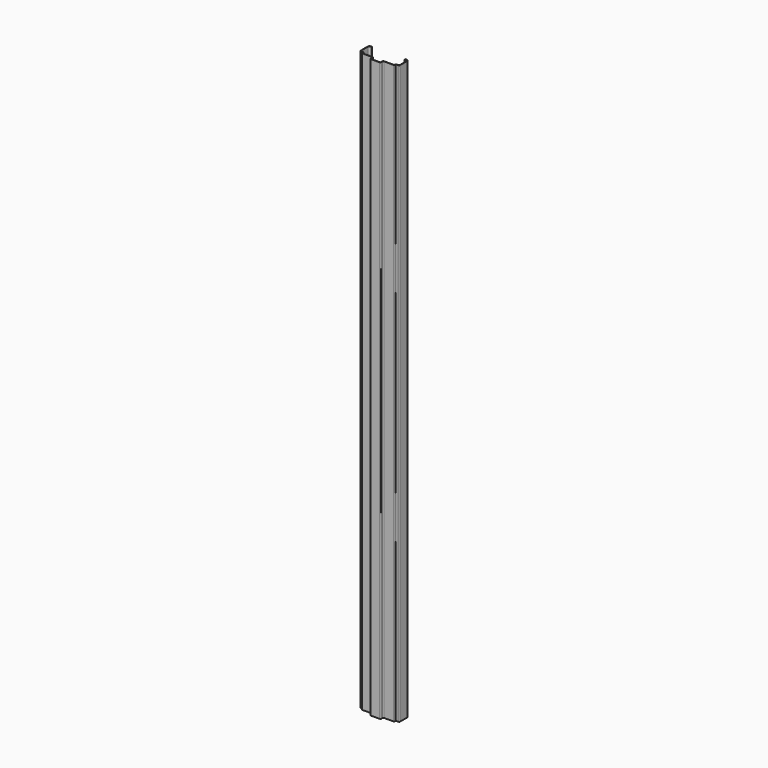
from build123d import *

# Parameters (mm, degrees)
F1_DEPTH     = 2070
F2_T1_DEPTH  = 2070
F2_T3_DEPTH  = 2070
F2_T5_DEPTH  = 2070
F2_T7_DEPTH  = 2070
F2_T9_DEPTH  = 2070
F2_T11_DEPTH = 2070
F2_T13_DEPTH = 2070
F2_T15_DEPTH = 2070
F2_T17_DEPTH = 2070
F2_T19_DEPTH = 2070
F2_T21_DEPTH = 2070
F2_T23_DEPTH = 2070
F2_T25_DEPTH = 2085
F2_T27_DEPTH = 2085
F2_T29_DEPTH = 2085
F2_T31_DEPTH = 2085
F2_T33_DEPTH = 2085
F2_T35_DEPTH = 2085
F2_T37_DEPTH = 2085
F2_T39_DEPTH = 2085
F2_T41_DEPTH = 2085
F2_T43_DEPTH = 2085
F2_T45_DEPTH = 2085
F2_T47_DEPTH = 2085
F3_R         = 5


# Not quite as in the source:
# - a fillet or chamfer that OpenCascade refuses, or shapes differently, is made with other operations: its cross-section is extruded or revolved along the edge and cut away or added


with BuildPart() as f1:
    # F0 (on Top) → F1 (new body)
    with BuildSketch(Plane.XY):
        Polygon((-18.5, 0), (0, 0), (18.5, 0), (18.5, 12), (58.5, 12), (58.5, 19), (70.5, 19), (70.5, 60), (58.5, 60), (58.5, 57), (59.5, 57), (59.5, 59), (69.5, 59), (69.5, 20), (57.5, 20), (57.5, 13), (17.5, 13), (17.5, 1), (0, 1), (-17.5, 1), (-17.5, 13), (-57.5, 13), (-57.5, 20), (-69.5, 20), (-69.5, 59), (-59.5, 59), (-59.5, 57), (-58.5, 57), (-58.5, 60), (-70.5, 60), (-70.5, 19), (-58.5, 19), (-58.5, 12), (-18.5, 12), align=None)
    extrude(amount=F1_DEPTH)

    # F2: fillet of radius 3 on 24 edges, made by hand

    # F2_s2 → F2_t1 (join)
    with BuildSketch(Plane.XY):
        with BuildLine():
            add(Edge.make_bspline(
                [(-21.5, 12), (-18.5, 12), (-18.5, 9)],
                knots=[0, 0, 0, 1, 1, 1], degree=2, weights=[1, 1, 1]))
            Line((-18.5, 9), (-18.5, 12))
            Line((-18.5, 12), (-21.5, 12))
        make_face()
    extrude(amount=F2_T1_DEPTH)

    # F2_s4 → F2_t3 (join)
    with BuildSketch(Plane.XY):
        with BuildLine():
            add(Edge.make_bspline(
                [(-61.5, 19), (-58.5, 19), (-58.5, 16)],
                knots=[0, 0, 0, 1, 1, 1], degree=2, weights=[1, 1, 1]))
            Line((-58.5, 16), (-58.5, 19))
            Line((-58.5, 19), (-61.5, 19))
        make_face()
    extrude(amount=F2_T3_DEPTH)

    # F2_s6 → F2_t5 (join)
    with BuildSketch(Plane.XY):
        with BuildLine():
            add(Edge.make_bspline(
                [(-62.3284271247, 59), (-60.2071067812, 59), (-59.5, 57)],
                knots=[0, 0, 0, 1, 1, 1], degree=2, weights=[1, 1, 1]))
            Line((-59.5, 57), (-59.5, 59))
            Line((-59.5, 59), (-62.3284271247, 59))
        make_face()
    extrude(amount=F2_T5_DEPTH)

    # F2_s8 → F2_t7 (join)
    with BuildSketch(Plane.XY):
        with BuildLine():
            add(Edge.make_bspline(
                [(-66.5, 20), (-69.5, 20), (-69.5, 23)],
                knots=[0, 0, 0, 1, 1, 1], degree=2, weights=[1, 1, 1]))
            Line((-69.5, 23), (-69.5, 20))
            Line((-69.5, 20), (-66.5, 20))
        make_face()
    extrude(amount=F2_T7_DEPTH)

    # F2_s10 → F2_t9 (join)
    with BuildSketch(Plane.XY):
        with BuildLine():
            add(Edge.make_bspline(
                [(-54.5, 13), (-57.5, 13), (-57.5, 16)],
                knots=[0, 0, 0, 1, 1, 1], degree=2, weights=[1, 1, 1]))
            Line((-57.5, 16), (-57.5, 13))
            Line((-57.5, 13), (-54.5, 13))
        make_face()
    extrude(amount=F2_T9_DEPTH)

    # F2_s12 → F2_t11 (join)
    with BuildSketch(Plane.XY):
        with BuildLine():
            add(Edge.make_bspline(
                [(-14.5, 1), (-17.5, 1), (-17.5, 4)],
                knots=[0, 0, 0, 1, 1, 1], degree=2, weights=[1, 1, 1]))
            Line((-17.5, 4), (-17.5, 1))
            Line((-17.5, 1), (-14.5, 1))
        make_face()
    extrude(amount=F2_T11_DEPTH)

    # F2_s14 → F2_t13 (join)
    with BuildSketch(Plane.XY):
        with BuildLine():
            add(Edge.make_bspline(
                [(17.5, 4), (17.5, 1), (14.5, 1)],
                knots=[0, 0, 0, 1, 1, 1], degree=2, weights=[1, 1, 1]))
            Line((14.5, 1), (17.5, 1))
            Line((17.5, 1), (17.5, 4))
        make_face()
    extrude(amount=F2_T13_DEPTH)

    # F2_s16 → F2_t15 (join)
    with BuildSketch(Plane.XY):
        with BuildLine():
            add(Edge.make_bspline(
                [(57.5, 16), (57.5, 13), (54.5, 13)],
                knots=[0, 0, 0, 1, 1, 1], degree=2, weights=[1, 1, 1]))
            Line((54.5, 13), (57.5, 13))
            Line((57.5, 13), (57.5, 16))
        make_face()
    extrude(amount=F2_T15_DEPTH)

    # F2_s18 → F2_t17 (join)
    with BuildSketch(Plane.XY):
        with BuildLine():
            add(Edge.make_bspline(
                [(69.5, 23), (69.5, 20), (66.5, 20)],
                knots=[0, 0, 0, 1, 1, 1], degree=2, weights=[1, 1, 1]))
            Line((66.5, 20), (69.5, 20))
            Line((69.5, 20), (69.5, 23))
        make_face()
    extrude(amount=F2_T17_DEPTH)

    # F2_s20 → F2_t19 (join)
    with BuildSketch(Plane.XY):
        with BuildLine():
            add(Edge.make_bspline(
                [(59.5, 57), (60.2071067812, 59), (62.3284271247, 59)],
                knots=[0, 0, 0, 1, 1, 1], degree=2, weights=[1, 1, 1]))
            Line((62.3284271247, 59), (59.5, 59))
            Line((59.5, 59), (59.5, 57))
        make_face()
    extrude(amount=F2_T19_DEPTH)

    # F2_s22 → F2_t21 (join)
    with BuildSketch(Plane.XY):
        with BuildLine():
            add(Edge.make_bspline(
                [(58.5, 16), (58.5, 19), (61.5, 19)],
                knots=[0, 0, 0, 1, 1, 1], degree=2, weights=[1, 1, 1]))
            Line((61.5, 19), (58.5, 19))
            Line((58.5, 19), (58.5, 16))
        make_face()
    extrude(amount=F2_T21_DEPTH)

    # F2_s24 → F2_t23 (join)
    with BuildSketch(Plane.XY):
        with BuildLine():
            add(Edge.make_bspline(
                [(18.5, 9), (18.5, 12), (21.5, 12)],
                knots=[0, 0, 0, 1, 1, 1], degree=2, weights=[1, 1, 1]))
            Line((21.5, 12), (18.5, 12))
            Line((18.5, 12), (18.5, 9))
        make_face()
    extrude(amount=F2_T23_DEPTH)

    # F2_s26 → F2_t25 (cut)
    with BuildSketch(Plane.XY.offset(-7.5)):
        with BuildLine():
            add(Edge.make_bspline(
                [(-15.5, 0), (-18.5, 0), (-18.5, 3)],
                knots=[0, 0, 0, 1, 1, 1], degree=2, weights=[1, 1, 1]))
            Line((-18.5, 3), (-18.5, 0))
            Line((-18.5, 0), (-15.5, 0))
        make_face()
    extrude(amount=F2_T25_DEPTH, mode=Mode.SUBTRACT)

    # F2_s28 → F2_t27 (cut)
    with BuildSketch(Plane.XY.offset(-7.5)):
        with BuildLine():
            add(Edge.make_bspline(
                [(15.5, 0), (18.5, 0), (18.5, 3)],
                knots=[0, 0, 0, 1, 1, 1], degree=2, weights=[1, 1, 1]))
            Line((18.5, 3), (18.5, 0))
            Line((18.5, 0), (15.5, 0))
        make_face()
    extrude(amount=F2_T27_DEPTH, mode=Mode.SUBTRACT)

    # F2_s30 → F2_t29 (cut)
    with BuildSketch(Plane.XY.offset(-7.5)):
        with BuildLine():
            add(Edge.make_bspline(
                [(-55.5, 12), (-58.5, 12), (-58.5, 15)],
                knots=[0, 0, 0, 1, 1, 1], degree=2, weights=[1, 1, 1]))
            Line((-58.5, 15), (-58.5, 12))
            Line((-58.5, 12), (-55.5, 12))
        make_face()
    extrude(amount=F2_T29_DEPTH, mode=Mode.SUBTRACT)

    # F2_s32 → F2_t31 (cut)
    with BuildSketch(Plane.XY.offset(-7.5)):
        with BuildLine():
            add(Edge.make_bspline(
                [(-67.5, 19), (-70.5, 19), (-70.5, 22)],
                knots=[0, 0, 0, 1, 1, 1], degree=2, weights=[1, 1, 1]))
            Line((-70.5, 22), (-70.5, 19))
            Line((-70.5, 19), (-67.5, 19))
        make_face()
    extrude(amount=F2_T31_DEPTH, mode=Mode.SUBTRACT)

    # F2_s34 → F2_t33 (cut)
    with BuildSketch(Plane.XY.offset(-7.5)):
        with BuildLine():
            add(Edge.make_bspline(
                [(-61.5, 60), (-58.5, 60), (-58.5, 57)],
                knots=[0, 0, 0, 1, 1, 1], degree=2, weights=[1, 1, 1]))
            Line((-58.5, 57), (-58.5, 60))
            Line((-58.5, 60), (-61.5, 60))
        make_face()
    extrude(amount=F2_T33_DEPTH, mode=Mode.SUBTRACT)

    # F2_s36 → F2_t35 (cut)
    with BuildSketch(Plane.XY.offset(-7.5)):
        with BuildLine():
            add(Edge.make_bspline(
                [(-60.5, 20), (-57.5, 20), (-57.5, 17)],
                knots=[0, 0, 0, 1, 1, 1], degree=2, weights=[1, 1, 1]))
            Line((-57.5, 17), (-57.5, 20))
            Line((-57.5, 20), (-60.5, 20))
        make_face()
    extrude(amount=F2_T35_DEPTH, mode=Mode.SUBTRACT)

    # F2_s38 → F2_t37 (cut)
    with BuildSketch(Plane.XY.offset(-7.5)):
        with BuildLine():
            add(Edge.make_bspline(
                [(-20.5, 13), (-17.5, 13), (-17.5, 10)],
                knots=[0, 0, 0, 1, 1, 1], degree=2, weights=[1, 1, 1]))
            Line((-17.5, 10), (-17.5, 13))
            Line((-17.5, 13), (-20.5, 13))
        make_face()
    extrude(amount=F2_T37_DEPTH, mode=Mode.SUBTRACT)

    # F2_s40 → F2_t39 (cut)
    with BuildSketch(Plane.XY.offset(-7.5)):
        with BuildLine():
            add(Edge.make_bspline(
                [(17.5, 10), (17.5, 13), (20.5, 13)],
                knots=[0, 0, 0, 1, 1, 1], degree=2, weights=[1, 1, 1]))
            Line((20.5, 13), (17.5, 13))
            Line((17.5, 13), (17.5, 10))
        make_face()
    extrude(amount=F2_T39_DEPTH, mode=Mode.SUBTRACT)

    # F2_s42 → F2_t41 (cut)
    with BuildSketch(Plane.XY.offset(-7.5)):
        with BuildLine():
            add(Edge.make_bspline(
                [(57.5, 17), (57.5, 20), (60.5, 20)],
                knots=[0, 0, 0, 1, 1, 1], degree=2, weights=[1, 1, 1]))
            Line((60.5, 20), (57.5, 20))
            Line((57.5, 20), (57.5, 17))
        make_face()
    extrude(amount=F2_T41_DEPTH, mode=Mode.SUBTRACT)

    # F2_s44 → F2_t43 (cut)
    with BuildSketch(Plane.XY.offset(-7.5)):
        with BuildLine():
            add(Edge.make_bspline(
                [(58.5, 57), (58.5, 60), (61.5, 60)],
                knots=[0, 0, 0, 1, 1, 1], degree=2, weights=[1, 1, 1]))
            Line((61.5, 60), (58.5, 60))
            Line((58.5, 60), (58.5, 57))
        make_face()
    extrude(amount=F2_T43_DEPTH, mode=Mode.SUBTRACT)

    # F2_s46 → F2_t45 (cut)
    with BuildSketch(Plane.XY.offset(-7.5)):
        with BuildLine():
            add(Edge.make_bspline(
                [(70.5, 22), (70.5, 19), (67.5, 19)],
                knots=[0, 0, 0, 1, 1, 1], degree=2, weights=[1, 1, 1]))
            Line((67.5, 19), (70.5, 19))
            Line((70.5, 19), (70.5, 22))
        make_face()
    extrude(amount=F2_T45_DEPTH, mode=Mode.SUBTRACT)

    # F2_s48 → F2_t47 (cut)
    with BuildSketch(Plane.XY.offset(-7.5)):
        with BuildLine():
            add(Edge.make_bspline(
                [(58.5, 15), (58.5, 12), (55.5, 12)],
                knots=[0, 0, 0, 1, 1, 1], degree=2, weights=[1, 1, 1]))
            Line((55.5, 12), (58.5, 12))
            Line((58.5, 12), (58.5, 15))
        make_face()
    extrude(amount=F2_T47_DEPTH, mode=Mode.SUBTRACT)

    # F3
    f3_edges = [f1.edges().sort_by_distance(p)[0] for p in [
        (-70.5, 60, 1035),
        (-69.5, 59, 1035),
        (70.5, 60, 1035),
        (69.5, 59, 1035),
    ]]
    fillet(f3_edges, radius=F3_R)


solid = f1.part
